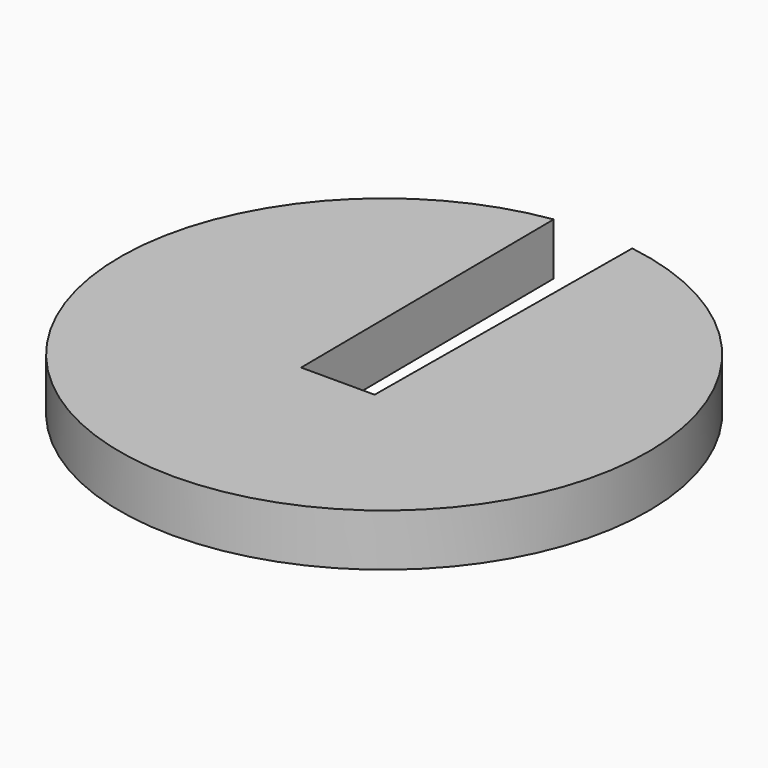
from build123d import *

# Parameters (mm, degrees)
F3_DEPTH = 3.81


# Not quite as in the source:
# - the program builds the solid bodies; features that only make, move or delete a surface that nothing else refers to are left out


with BuildPart() as f3:
    # F1 (on Top) → F3 (new body)
    with BuildSketch(Plane.XY):
        with BuildLine():
            Line((-2.684316365, -18.0109087378), (-2.870472083, 5.2918509166))
            ThreePointArc((-2.870472083, 5.2918509166), (0, -33.0777025508), (2.870472083, 5.2918509166))
            Line((2.870472083, 5.2918509166), (2.6843168307, -18.0109087378))
            Line((2.6843168307, -18.0109087378), (-2.684316365, -18.0109087378))
        make_face()
    extrude(amount=F3_DEPTH)


solid = f3.part
